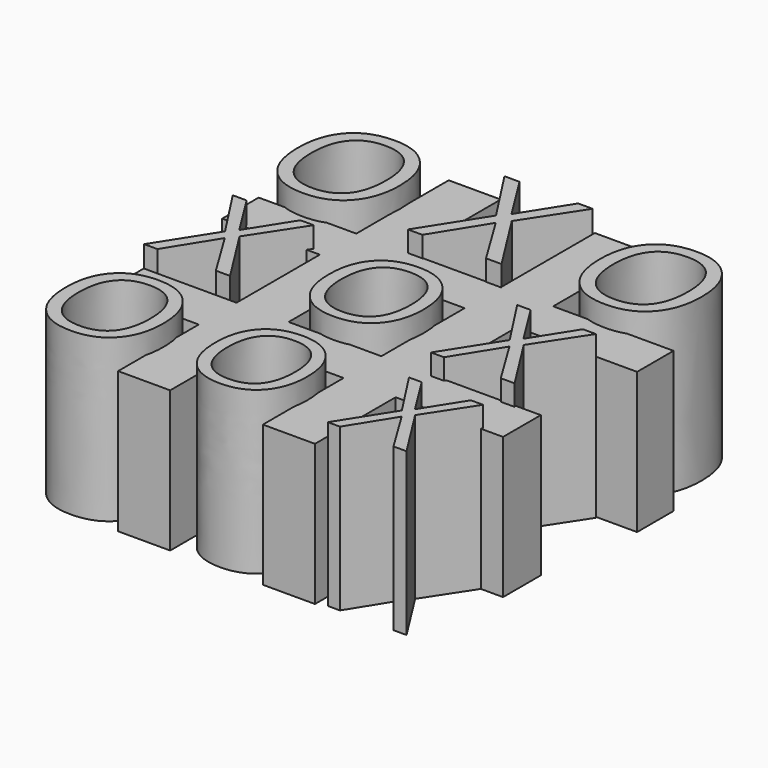
from build123d import *

# Parameters (mm, degrees)
F0_W           = 3.1874514517
F0_H           = 7.0721568715
F0_H_2         = 2.7890200551
F0_W_2         = 5.9764698337
F0_W_3         = 5.6776478199
F0_H_3         = 6.3749020669
F0_W_4         = 3.1874503363
F0_H_4         = 7.1717640235
F0_H_5         = 2.888627486
F0_W_5         = 5.6776472622
F0_W_6         = 7.3709805584
F0_H_6         = 6.1756863686
F0_W_7         = 6.5741177652
F1_DEPTH       = 8.636
F2_TEXT_SIZE   = 10.0699337458
F2_TEXT_SIZE_2 = 9.5181574579
F2_TEXT_SIZE_3 = 9.2443478126
F2_TEXT_SIZE_4 = 8.8537415852
F2_TEXT_SIZE_5 = 8.9839437149
F2_TEXT_SIZE_6 = 9.1141458446
F2_TEXT_SIZE_7 = 8.5933379725
F2_TEXT_SIZE_8 = 8.4631351961
F2_TEXT_SIZE_9 = 9.5047522336
F3_DEPTH       = 9.906


# Not quite as in the source:
# - Text() gives the source's letters only with a copy of the font that has no kerning and outlines rounded to 1/6400 em; it was checked with that copy


with BuildPart() as f1:
    # F0 (on Top) → F1 (new body)
    with BuildSketch(Plane.XY):
        with Locations((-6.3947822173, 7.5672450385)):
            Rectangle(F0_W, F0_H)
        with Locations((-6.3947822173, 2.6366565752)):
            Rectangle(F0_W, F0_H_2)
        with Locations((-10.97674286, 2.6366565752)):
            Rectangle(F0_W_2, F0_H_2)
        with Locations((-1.9622325815, 2.6366565752)):
            Rectangle(F0_W_3, F0_H_2)
        with Locations((-6.3947822173, -1.9453044858)):
            Rectangle(F0_W, F0_H_3)
        with Locations((2.4703164966, 2.6366565752)):
            Rectangle(F0_W_4, F0_H_2)
        with Locations((2.4703164966, 7.6170486145)):
            Rectangle(F0_W_4, F0_H_4)
        with Locations((-6.3947822173, -6.5770692622)):
            Rectangle(F0_W, F0_H_5)
        with Locations((-10.8273315743, -6.5770692622)):
            Rectangle(F0_W_5, F0_H_5)
        with Locations((-1.9622325815, -6.5770692622)):
            Rectangle(F0_W_3, F0_H_5)
        with Locations((2.4703164966, -1.9453044858)):
            Rectangle(F0_W_4, F0_H_3)
        with Locations((7.7495319439, 2.6366565752)):
            Rectangle(F0_W_6, F0_H_2)
        with Locations((-6.3947822173, -11.1092261895)):
            Rectangle(F0_W, F0_H_6)
        with Locations((2.4703164966, -6.5770692622)):
            Rectangle(F0_W_4, F0_H_5)
        with Locations((2.4703164966, -11.1092261895)):
            Rectangle(F0_W_4, F0_H_6)
        with Locations((7.3511005473, -6.5770692622)):
            Rectangle(F0_W_7, F0_H_5)
    extrude(amount=F1_DEPTH)

    # F2 (on Top) → F3 (join)
    with BuildSketch(Plane.XY):
        with Locations((-4.8474273644, 4.0034209378)):
            Text('X', F2_TEXT_SIZE, font='Open Sans', text_align=(TextAlign.LEFT, TextAlign.BOTTOM))
        with Locations((-14.7794177756, 3.9041002747)):
            Text('O', F2_TEXT_SIZE_2, font='Open Sans', text_align=(TextAlign.LEFT, TextAlign.BOTTOM))
        with Locations((-13.7402471155, -5.062198732)):
            Text('X', F2_TEXT_SIZE_3, font='Open Sans', text_align=(TextAlign.LEFT, TextAlign.BOTTOM))
        with Locations((-5.3968974389, -5.1559442654)):
            Text('O', F2_TEXT_SIZE_4, font='Open Sans', text_align=(TextAlign.LEFT, TextAlign.BOTTOM))
        with Locations((3.9776521735, -5.2496897988)):
            Text('X', F2_TEXT_SIZE_5, font='Open Sans', text_align=(TextAlign.LEFT, TextAlign.BOTTOM))
        with Locations((-14.3964653835, -14.1555117443)):
            Text('O', F2_TEXT_SIZE_6, font='Open Sans', text_align=(TextAlign.LEFT, TextAlign.BOTTOM))
        with Locations((-5.2094063722, -13.9680206776)):
            Text('O', F2_TEXT_SIZE_7, font='Open Sans', text_align=(TextAlign.LEFT, TextAlign.BOTTOM))
        with Locations((4.6338709071, -13.9680206776)):
            Text('X', F2_TEXT_SIZE_8, font='Open Sans', text_align=(TextAlign.LEFT, TextAlign.BOTTOM))
        with Locations((3.6964153405, 3.9373692125)):
            Text('O', F2_TEXT_SIZE_9, font='Open Sans', text_align=(TextAlign.LEFT, TextAlign.BOTTOM))
    extrude(amount=F3_DEPTH)


solid = f1.part
